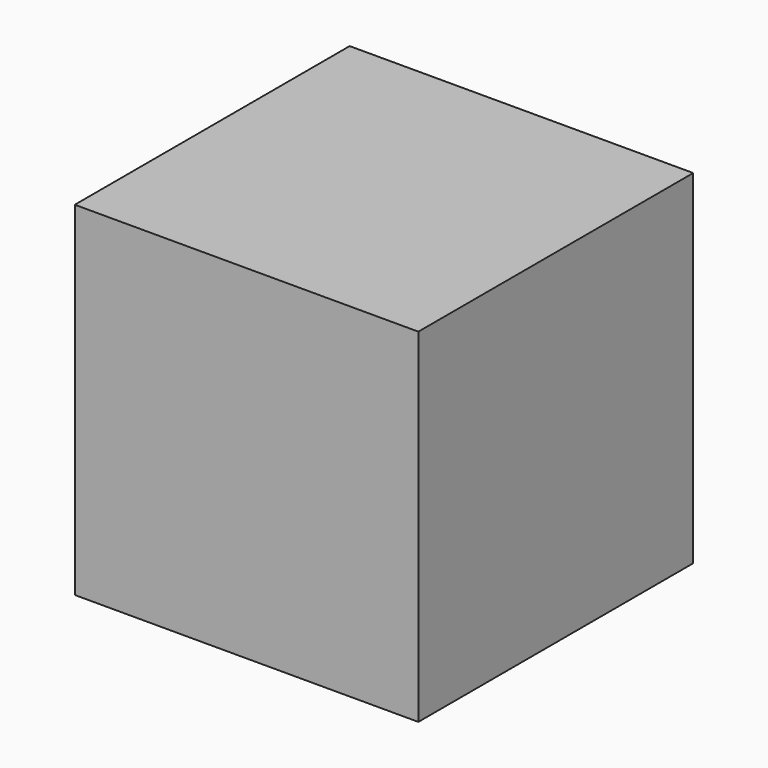
from build123d import *

# Parameters (mm, degrees)
F0_W     = 100
F0_H     = 100
F1_DEPTH = 100
F6_R     = 5
F7_DEPTH = 50.001


# Not quite as in the source:
# - a feature of the source that left no trace in its solid (it failed there, or was rolled back) is left out


with BuildPart() as f1:
    # F0 (on Front) → F1 (new body)
    with BuildSketch(Plane.XZ):
        Rectangle(F0_W, F0_H)
    extrude(amount=F1_DEPTH)

    # F6 (on Right) → F7 (cut, through all)
    with BuildSketch(Plane.YZ):
        with Locations((-17.9369883015, 0)):
            Circle(F6_R)
    extrude(amount=-F7_DEPTH, mode=Mode.SUBTRACT)


solid = f1.part
